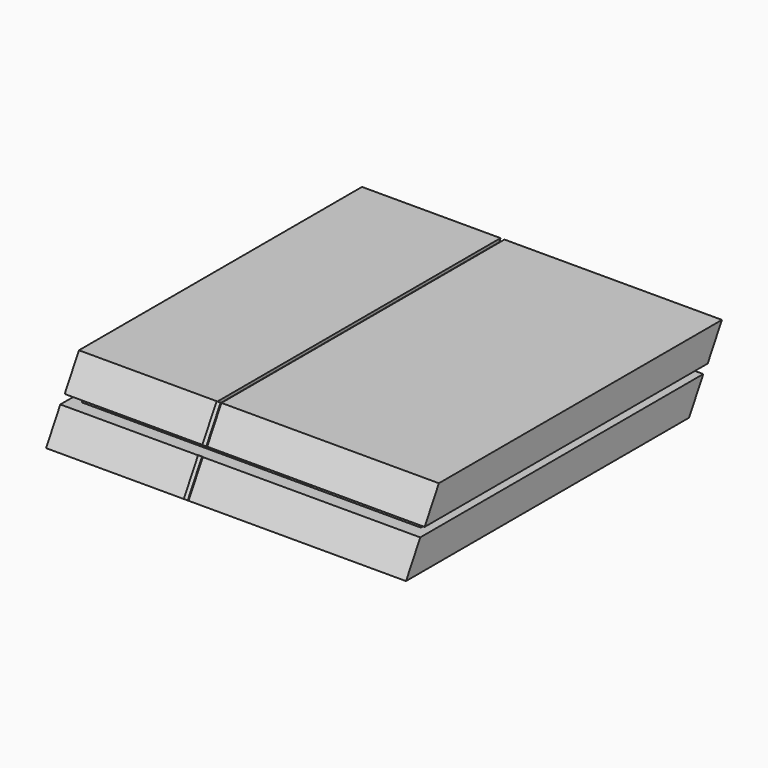
from build123d import *

# Parameters (mm, degrees)
F0_W         = 275.082
F0_H         = 305.054
F1_DEPTH     = 23.876
F2_T1_DEPTH  = 494.2621936506
F3_T1_DEPTH  = 494.2621936506
F4_W         = 259.08
F4_H         = 254.254
F5_DEPTH     = 5.334
F7_W         = 259.600803256
F7_H         = 19.5427685976
F8_DEPTH     = 2.54
F9_W         = 31.0830250382
F9_H         = 20.8677053452
F9_W_2       = 224.7763052583
F10_DEPTH    = 2.54
F12_W        = 2.999994
F12_H        = 274.32
F13_DEPTH    = 2.286
F14_W        = 2.999994
F14_H        = 27.4787114047
F15_DEPTH    = 1.016
F17_W        = 127.1692942828
F17_H        = 3.2591354102
F18_DEPTH    = 147.32
F19_W        = 12.3909562826
F19_H        = 3.428991884
F20_DEPTH    = 25.4
F21_W        = 12.3321115971
F21_H        = 3.3447202295
F22_DEPTH    = 25.4
F23_T1_DEPTH = 286.765919198


# Not quite as in the source:
# - a fillet or chamfer that OpenCascade refuses, or shapes differently, is made with other operations: its cross-section is extruded or revolved along the edge and cut away or added


with BuildPart() as f1:
    # F0 (on Top) → F1 (new body)
    with BuildSketch(Plane.XY):
        Rectangle(F0_W, F0_H)
    extrude(amount=F1_DEPTH)

    # F2: chamfer of 24.13 x 42.3559091851 on 1 edges, made by hand

    # F2_s2 → F2_t1 (cut)
    with BuildSketch(Plane.YZ.offset(-247.1310968253)):
        Polygon((-152.527, -18.4799091851), (-128.397, 23.876), (-152.527, 23.876), align=None)
    extrude(amount=F2_T1_DEPTH, mode=Mode.SUBTRACT)

    # F3: chamfer of 24.13 x 42.3559091851 on 1 edges, made by hand

    # F3_s2 → F3_t1 (cut)
    with BuildSketch(Plane.YZ.offset(-247.1310968253)):
        Polygon((152.527, 42.3559091851), (128.397, 0), (152.527, 0), align=None)
    extrude(amount=F3_T1_DEPTH, mode=Mode.SUBTRACT)


with BuildPart() as f5:
    # F4 (on face) → F5 (new body)
    with BuildSketch(Plane.XY.offset(23.876)):
        with Locations((0.4944914198, 8.7817526798)):
            Rectangle(F4_W, F4_H)
    extrude(amount=F5_DEPTH)

    # F17 (on face) → F18 (cut)
    with BuildSketch(Plane.XZ.offset(118.3452473202)):
        with Locations((-51.6607919708, 26.5423739329)):
            Rectangle(F17_W, F17_H)
    extrude(amount=-F18_DEPTH, mode=Mode.SUBTRACT)

    # F19 (on face) → F20 (cut)
    with BuildSketch(Plane.XZ.offset(118.3452473202)):
        with Locations((24.3740323931, 26.5821330249)):
            Rectangle(F19_W, F19_H)
    extrude(amount=-F20_DEPTH, mode=Mode.SUBTRACT)

    # F21 (on face) → F22 (cut)
    with BuildSketch(Plane.XZ.offset(118.3452473202)):
        with Locations((41.4287000895, 26.5834620222)):
            Rectangle(F21_W, F21_H)
    extrude(amount=-F22_DEPTH, mode=Mode.SUBTRACT)

    # F23: chamfer of 3.048 x 5.3502201076 on 1 edges, made by hand

    # F23_s2 → F23_t1 (cut)
    with BuildSketch(Plane.YZ.offset(-142.8884681792)):
        Polygon((132.8607526798, 23.876), (135.9087526798, 29.2262201076), (135.9087526798, 23.876), align=None)
    extrude(amount=F23_T1_DEPTH, mode=Mode.SUBTRACT)


with BuildPart() as f6_1:
    # F6: copy of F1
    add(f1.part.moved(Location((0, 17.78, 29.21))))

    # F7 (on face) → F8 (cut)
    with BuildSketch(Plane(origin=(0, 97.7960876904, -55.7140583539), x_dir=(-1, 0, 0), z_dir=(0, 0.8688908169, -0.4950037861))):
        with Locations((-1.2951269746, 110.8248233795)):
            Rectangle(F7_W, F7_H)
    extrude(amount=-F8_DEPTH, mode=Mode.SUBTRACT)

    # F12 (on face) → F13 (cut)
    with BuildSketch(Plane.XY.offset(53.086)):
        with Locations((-30.1378168959, 24.599660728)):
            Rectangle(F12_W, F12_H)
    extrude(amount=-F13_DEPTH, mode=Mode.SUBTRACT)


with BuildPart() as f1_1:
    add(f1.part)

    # F9 (on face) → F10 (cut)
    with BuildSketch(Plane(origin=(0, 96.9360438055, -55.2240946312), x_dir=(-1, 0, 0), z_dir=(0, 0.8688908169, -0.4950037861))):
        with Locations((-115.5540160835, 77.8000429273)):
            Rectangle(F9_W, F9_H)
        with Locations((16.1171220243, 77.8000429273)):
            Rectangle(F9_W_2, F9_H)
    extrude(amount=-F10_DEPTH, mode=Mode.SUBTRACT)


with BuildPart() as f15:
    # F14 (on face) → F15 (new body)
    with BuildSketch(Plane(origin=(0, -106.345168853, 60.5844373027), x_dir=(1, 0, 0), z_dir=(0, -0.8688908169, 0.4950037861))):
        with Locations((-30.1378168959, -22.3692516073)):
            Rectangle(F14_W, F14_H)
    extrude(amount=F15_DEPTH)


with BuildPart() as f16_1:
    # F16: copy of F15
    add(f15.part.moved(Location((0, -17.6784, -29.083))))


solid = Compound([f5.part, f6_1.part, f1_1.part, f15.part, f16_1.part])
